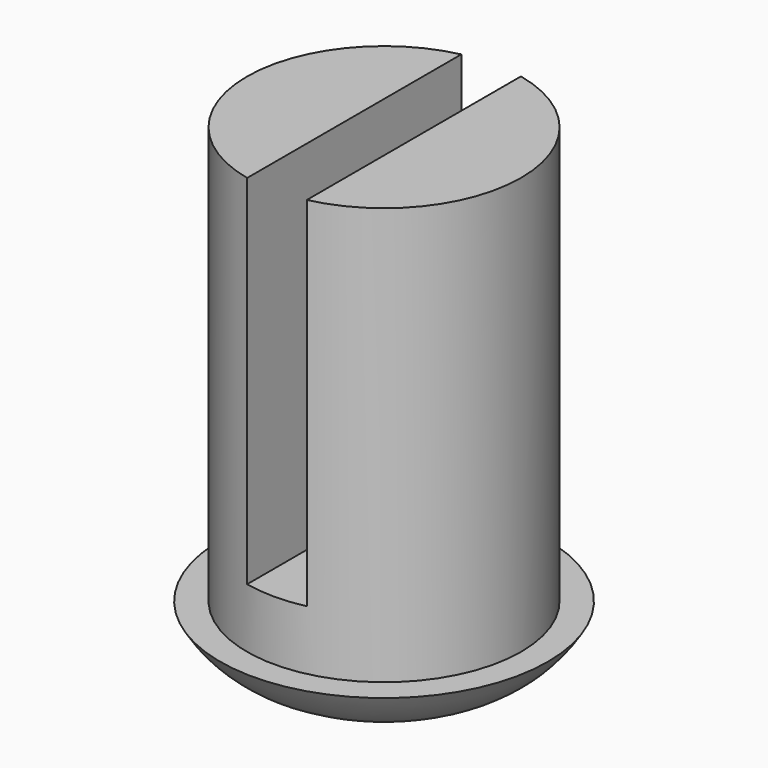
from build123d import *

# Parameters (mm, degrees)
F0_R     = 5.842
F1_DEPTH = 17.78
F3_DEPTH = 15.24
F4_R     = 6.985
F4_R_2   = 5.842
F5_DEPTH = 2.54


# Not quite as in the source:
# - a fillet or chamfer that OpenCascade refuses, or shapes differently, is made with other operations: its cross-section is extruded or revolved along the edge and cut away or added


with BuildPart() as f1:
    # F0 (on Top) → F1 (new body)
    with BuildSketch(Plane.XY):
        Circle(F0_R)
    extrude(amount=F1_DEPTH)

    # F2 (on face) → F3 (cut)
    with BuildSketch(Plane.XY.offset(17.78)):
        with BuildLine():
            Line((1.27, -5.7022858574), (1.27, 5.7022858574))
            ThreePointArc((1.27, 5.7022858574), (0, 5.842), (-1.27, 5.7022858574))
            Line((-1.27, 5.7022858574), (-1.27, -5.7022858574))
            ThreePointArc((-1.27, -5.7022858574), (0, -5.842), (1.27, -5.7022858574))
        make_face()
    extrude(amount=-F3_DEPTH, mode=Mode.SUBTRACT)

    # F4 (on face) → F5 (join)
    with BuildSketch(Plane(origin=(0, 0, 0), x_dir=(1, 0, 0), z_dir=(0, 0, -1))):
        Circle(F4_R)
        Circle(F4_R_2, mode=Mode.SUBTRACT)
        Circle(F4_R_2)
    extrude(amount=F5_DEPTH)

    # F6: fillet of radius 5.08 on 1 edges, made by hand

    # F6_s1 → F6_t2 (revolve, cut)
    with BuildSketch(Plane.XZ):
        with BuildLine():
            ThreePointArc((6.985, 0), (5.1255909488, -1.8594090512), (2.5855909488, -2.54))
            Line((2.5855909488, -2.54), (6.985, -2.54))
            Line((6.985, -2.54), (6.985, 0))
        make_face()
    revolve(axis=Axis((0, 0, -2.54), (0, 0, -1)), mode=Mode.SUBTRACT)


solid = f1.part
